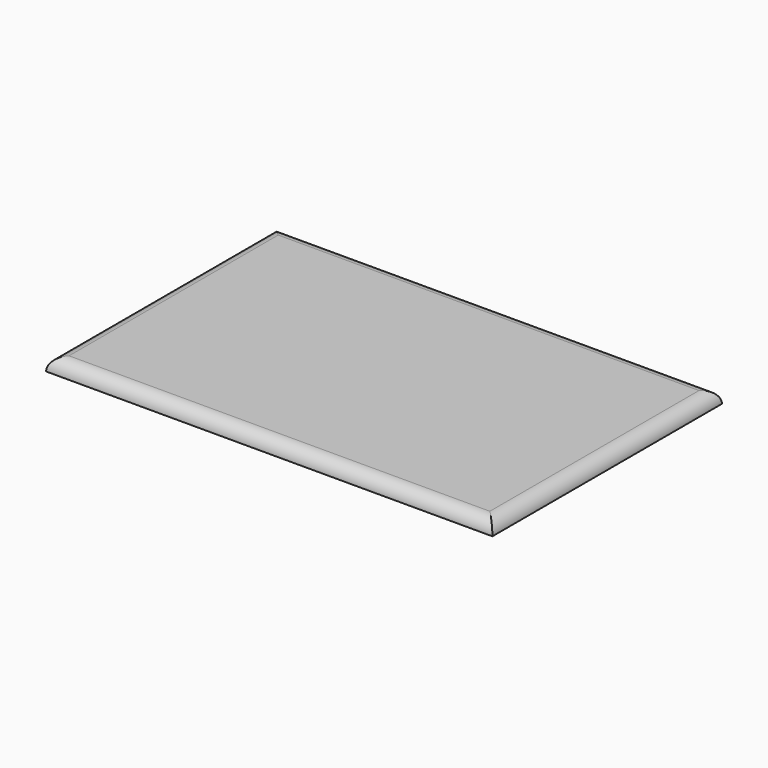
from build123d import *

# Parameters (mm, degrees)
F0_W     = 70
F0_H     = 45
F1_DEPTH = 2
F2_R     = 1.99999


# Not quite as in the source:
# - a fillet or chamfer is up to 0.001 mm smaller than in the source, because OpenCascade refuses the exact size


with BuildPart() as f1:
    # F0 (on Top) → F1 (new body)
    with BuildSketch(Plane.XY):
        with Locations((-29.475324953, 22.5)):
            Rectangle(F0_W, F0_H)
    extrude(amount=F1_DEPTH)

    # F2 (radius 2 in the source; OpenCascade refuses exactly that, so slightly less here)
    f2_edges = [f1.edges().sort_by_distance(p)[0] for p in [
        (5.524675, 22.5, 2),
        (-29.475325, 0, 2),
        (-64.475325, 22.5, 2),
        (-29.475325, 45, 2),
    ]]
    fillet(f2_edges, radius=F2_R)


solid = f1.part
